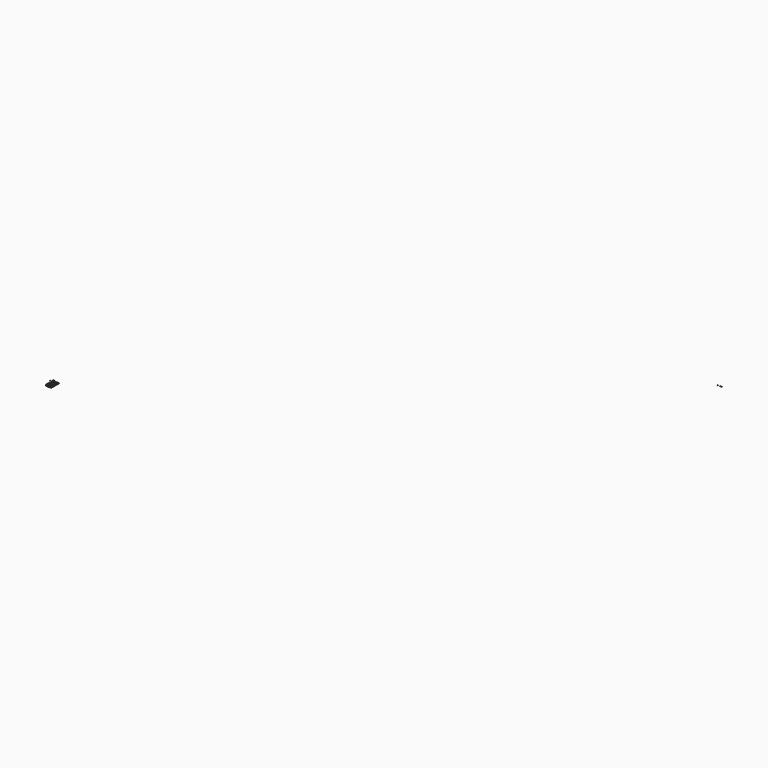
from build123d import *

# Parameters (mm, degrees)
F1_DEPTH  = 25.4
F2_T      = -2.54
F3_W      = 9.5226986027
F3_H      = 10.3040856934
F3_H_2    = 9.245954237
F3_W_2    = 10.041333518
F4_DEPTH  = 96.52
F5_W      = 9.5226986027
F5_H      = 10.1391447401
F5_H_2    = 9.4019619441
F6_DEPTH  = 193.04
F7_W      = 9.5582157373
F7_H      = 8.6707919836
F9_DEPTH  = 85.344
F10_SIZE  = 5.08
F11_W     = 10.0838167286
F11_H     = 10.4020283642
F12_DEPTH = 22.86
F13_W     = 1.6963680973
F13_H     = 7.6626996374
F14_DEPTH = 401.828
F15_W     = 1.4758335733
F15_H     = 7.6626996374
F16_DEPTH = 330.7588
F17_W     = 1.560665884
F17_H     = 7.6605677605
F18_DEPTH = 324.866
F19_W     = 9.5226986027
F19_H     = 9.3857411835
F19_H_2   = 9.4867787715
F19_W_2   = 9.1516710818
F19_H_3   = 9.245954237
F20_DEPTH = 96.52
F21_W     = 103.7419562926
F21_H     = 195.58
F22_DEPTH = 5.334
F23_W     = 90.4028788209
F23_H     = 111.0128611326
F24_DEPTH = 7.366
F25_W     = 37.6309305429
F25_H     = 49.3094902486
F25_W_2   = 37.3065290041
F25_H_2   = 49.6338959783
F26_DEPTH = 5.08
F29_R     = 2.0259765458
F30_DEPTH = 291.592
F31_R     = 3.4647538712
F32_DEPTH = 380.492
F33_R     = 1.8315999193
F34_DEPTH = 290.322


# Not quite as in the source:
# - the program builds the solid bodies; features that only make, move or delete a surface that nothing else refers to are left out


with BuildPart() as f1:
    # F0 (on Top) → F1 (new body)
    with BuildSketch(Plane.XY):
        Polygon((-124.2847517133, -35.648856312), (-174.5952665806, -35.648856312), (-174.5952665806, -369.8091506958), (230.7426333427, -369.8091506958), (230.7426333427, 394.0069079399), (-174.5952665806, 394.0069079399), (-174.5952665806, 63.9014318585), (-124.2847517133, 63.9014318585), (-124.2847517133, 322.5328326225), (-72.0331966877, 322.5328326225), (-72.0331966877, 65.4967414162), (5.2474793047, 63.9014318585), (5.2474793047, 323.4679299602), (50.5458692184, 322.5328326225), (50.5458692184, 63.9014318585), (126.9210129976, 63.9014318585), (126.9210129976, 322.5328326225), (179.8037737608, 322.5328326225), (179.8037737608, -289.8495197296), (126.9210129976, -289.8495197296), (126.9210129976, -35.648856312), (50.5458692184, -35.648856312), (50.5458692184, -290.8929410925), (0, -289.8495197296), (5.2474793047, -35.648856312), (-72.0331966877, -35.648856312), (-72.0331966877, -289.8495197296), (-124.2847517133, -289.8495197296), align=None)
    extrude(amount=F1_DEPTH)

    # F2
    f2_openings = [f1.faces().sort_by_distance(p)[0] for p in [
        (-132.931796, -162.749188, 25.4),
    ]]
    offset(amount=F2_T, openings=f2_openings, kind=Kind.INTERSECTION)

    # F3 (on face) → F4 (join)
    with BuildSketch(Plane.XY.offset(2.54)):
        with Locations((-167.2939172792, 386.3148650932)):
            Rectangle(F3_W, F3_H)
        with Locations((-167.2939172792, -362.6461735773)):
            Rectangle(F3_W, F3_H_2)
        with Locations((223.1819665837, -362.6461735773)):
            Rectangle(F3_W_2, F3_H_2)
    extrude(amount=F4_DEPTH)

    # F5 (on face) → F6 (join)
    with BuildSketch(Plane.XY.offset(2.54)):
        with Locations((-167.2939172792, 71.5110042286)):
            Rectangle(F5_W, F5_H)
        with Locations((-167.2939172792, -42.8898372841)):
            Rectangle(F5_W, F5_H_2)
    extrude(amount=F6_DEPTH)


with BuildPart() as f1_1:
    # F8: moved
    add(f1.part.moved(Location((0, -13.716, 0))))

    # F11 (on face) → F12 (join)
    with BuildSketch(Plane.XY.offset(2.54)):
        with Locations((223.1607249784, 372.5498937578)):
            Rectangle(F11_W, F11_H)
    extrude(amount=F12_DEPTH)

    # F13 (on face) → F14 (join)
    with BuildSketch(Plane(origin=(-172.0552665806, 0, 0), x_dir=(0, -1, 0), z_dir=(-1, 0, 0))):
        with Locations((381.8333347445, 95.2286501813)):
            Rectangle(F13_W, F13_H)
    extrude(amount=-F14_DEPTH)

    # F15 (on face) → F16 (join)
    with BuildSketch(Plane.XZ.offset(382.6815187931)):
        with Locations((-172.7931833673, 95.2286501813)):
            Rectangle(F15_W, F15_H)
    extrude(amount=-F16_DEPTH)

    # F17 (on face) → F18 (join)
    with BuildSketch(Plane.XZ.offset(-52.7254318585)):
        with Locations((-172.8355995226, 95.2429324389)):
            Rectangle(F17_W, F17_H)
    extrude(amount=-F18_DEPTH)

    # F19 (on face) → F20 (join)
    with BuildSketch(Plane.XY.offset(2.54)):
        with Locations((-167.2939172792, 219.8485700144)):
            Rectangle(F19_W, F19_H)
        with Locations((-167.2939172792, -221.2663967432)):
            Rectangle(F19_W, F19_H_2)
        with Locations((32.3902014643, -376.3621735773)):
            Rectangle(F19_W_2, F19_H_3)
    extrude(amount=F20_DEPTH)

    # F29 (on face) → F30 (join)
    with BuildSketch(Plane(origin=(1.0377747393, 50.2723330385, 0), x_dir=(0.9997870001, -0.0206386621, 0), z_dir=(-0.0206386621, -0.9997870001, 0))):
        with Locations((-34.2426486313, 25.9369704872)):
            Circle(F29_R)
    extrude(amount=-F30_DEPTH)

    # F31 (on face) → F32 (join)
    with BuildSketch(Plane.YZ.offset(-172.0552665806)):
        with Locations((343.0432975292, 25.4)):
            Circle(F31_R)
    extrude(amount=F32_DEPTH)

    # F33 (on face) → F34 (join)
    with BuildSketch(Plane(origin=(0, 52.7254318585, 0), x_dir=(-1, 0, 0), z_dir=(0, 1, 0))):
        with Locations((-88.733441108, 25.4)):
            Circle(F33_R)
    extrude(amount=F34_DEPTH)


with BuildPart() as f9:
    # F7 (on Front) → F9 (new body, symmetric)
    with BuildSketch(Plane.XZ):
        with Locations((-167.2844663262, 199.9216154218)):
            Rectangle(F7_W, F7_H)
    extrude(amount=F9_DEPTH, both=True)

    # F10
    f10_edges = [f9.edges().sort_by_distance(p)[0] for p in [
        (-167.284466, 85.344, 195.586219),
        (-167.284466, -85.344, 195.586219),
    ]]
    chamfer(f10_edges, length=F10_SIZE)


with BuildPart() as f22:
    # F21 (on face) → F22 (new body)
    with BuildSketch(Plane(origin=(-172.0552665806, 0, 0), x_dir=(0, -1, 0), z_dir=(-1, 0, 0))):
        with Locations((-0.8544537122, 97.79)):
            Rectangle(F21_W, F21_H)
    extrude(amount=-F22_DEPTH)

    # F23 (on face) → F24 (cut)
    with BuildSketch(Plane(origin=(-172.0552665806, 0, 0), x_dir=(0, -1, 0), z_dir=(-1, 0, 0))):
        with Locations((-1.2207254767, 134.5460042357)):
            Rectangle(F23_W, F23_H)
    extrude(amount=-F24_DEPTH, mode=Mode.SUBTRACT)

    # F25 (on face) → F26 (cut)
    with BuildSketch(Plane(origin=(-172.0552665806, 0, 0), x_dir=(0, -1, 0), z_dir=(-1, 0, 0))):
        with Locations((-25.8872956038, 44.0689856187)):
            Rectangle(F25_W, F25_H)
        with Locations((24.8820164707, 44.2311884835)):
            Rectangle(F25_W_2, F25_H_2)
    extrude(amount=-F26_DEPTH, mode=Mode.SUBTRACT)


with BuildPart() as f32:
    # F31 (on face) → F32, piece 2 (new body)
    with BuildSketch(Plane.YZ.offset(-172.0552665806)):
        with Locations((66291.0308837891, -27038.0897521973)):
            Circle(F31_R)
    extrude(amount=F32_DEPTH)


solid = Compound([f1_1.part, f9.part, f22.part, f32.part])
